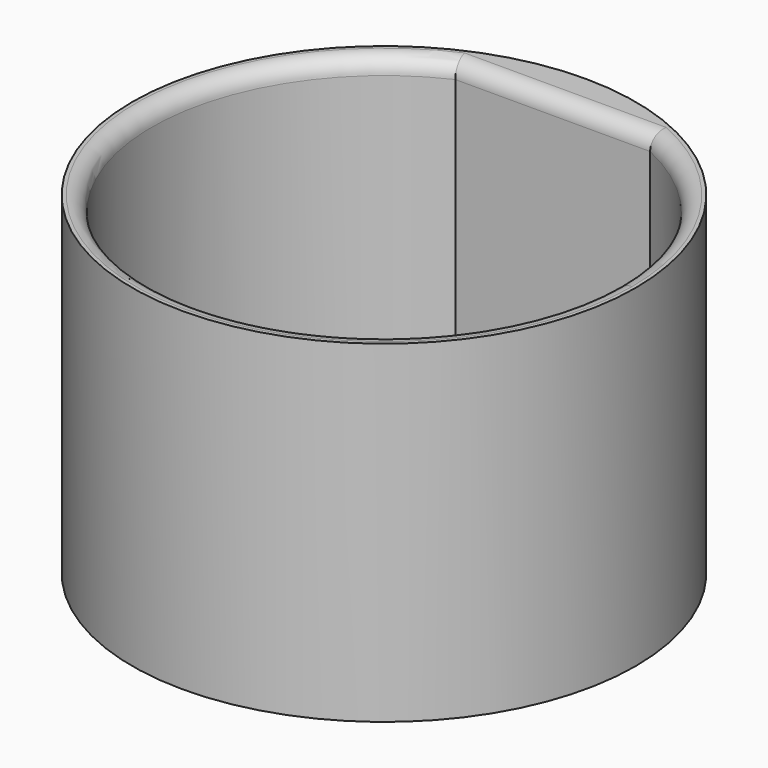
from build123d import *

# Parameters (mm, degrees)
F0_R     = 15.875
F1_DEPTH = 21
F2_R     = 1


# Not quite as in the source:
# - a feature names something its author has since deleted; it is built from what else it names


with BuildPart() as f1:
    # F0 (on Top) → F1 (new body)
    with BuildSketch(Plane.XY):
        Circle(F0_R)
        with BuildLine():
            ThreePointArc((6.1426785688, 13.3), (12.3412467165, 7.8940565924), (14.65, 0))
            ThreePointArc((14.65, 0), (-7.8940565924, -12.3412467165), (-6.1426785688, 13.3))
            ThreePointArc((-6.1426785688, 13.3), (0, 14.65), (6.1426785688, 13.3))
        make_face(mode=Mode.SUBTRACT)
        with BuildLine():
            Line((-6.1426785688, 13.3), (6.1426785688, 13.3))
            ThreePointArc((6.1426785688, 13.3), (0, 14.65), (-6.1426785688, 13.3))
        make_face()
    extrude(amount=F1_DEPTH)

    # F2
    f2_edges = [f1.edges().sort_by_distance(p)[0] for p in [
        (0, -14.65, 21),
        (0, 13.3, 21),
        (0, -14.65, 0),
        (0, 13.3, 0),
    ]]
    fillet(f2_edges, radius=F2_R)


solid = f1.part
